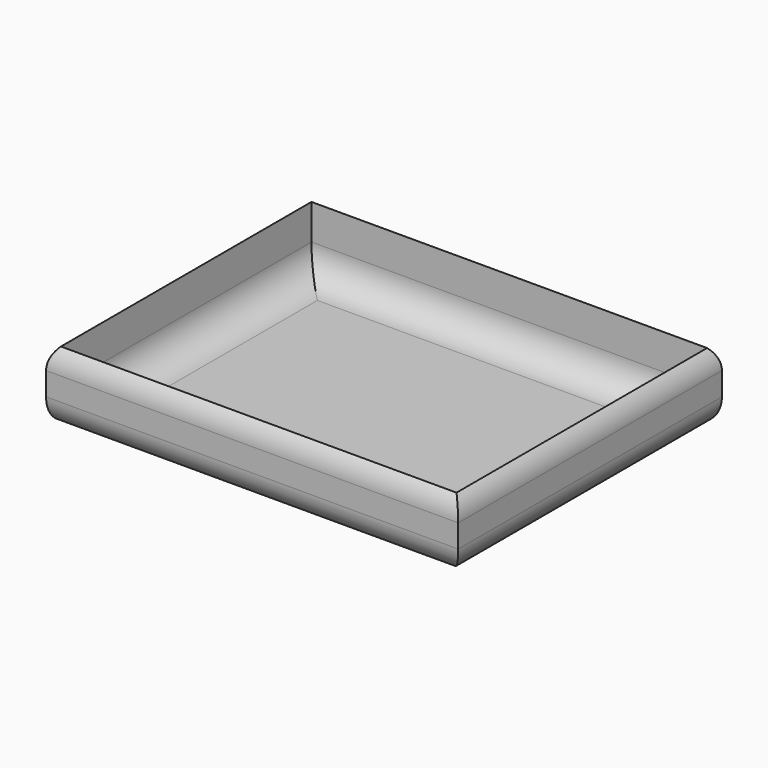
from build123d import *

# Parameters (mm, degrees)
F0_W        = 125
F0_H        = 100
F1_DEPTH    = 25
F2_T        = -2.5
F3_T1_DEPTH = 95
F3_T3_DEPTH = 120
F3_T5_DEPTH = 170
F3_T7_DEPTH = 145


# Not quite as in the source:
# - a fillet or chamfer that OpenCascade refuses, or shapes differently, is made with other operations: its cross-section is extruded or revolved along the edge and cut away or added


with BuildPart() as f1:
    # F0 (on Top) → F1 (new body)
    with BuildSketch(Plane.XY):
        with Locations((62.5, 50)):
            Rectangle(F0_W, F0_H)
    extrude(amount=F1_DEPTH)

    # F2
    f2_openings = [f1.faces().sort_by_distance(p)[0] for p in [
        (62.5, 50, 25),
    ]]
    offset(amount=F2_T, openings=f2_openings)

    # F3: fillet of radius 9 on 10 edges, made by hand

    # F3_s2 → F3_t1 (join)
    with BuildSketch(Plane.XZ.offset(-97.5)):
        with BuildLine():
            ThreePointArc((2.5, 11.5), (5.1360389693, 5.1360389693), (11.5, 2.5))
            Line((11.5, 2.5), (2.5, 2.5))
            Line((2.5, 2.5), (2.5, 11.5))
        make_face()
        with BuildLine():
            ThreePointArc((122.5, 11.5), (119.8639610307, 5.1360389693), (113.5, 2.5))
            Line((113.5, 2.5), (122.5, 2.5))
            Line((122.5, 2.5), (122.5, 11.5))
        make_face()
    extrude(amount=F3_T1_DEPTH)

    # F3_s4 → F3_t3 (join)
    with BuildSketch(Plane.YZ.offset(2.5)):
        with BuildLine():
            ThreePointArc((2.5, 11.5), (5.1360389693, 5.1360389693), (11.5, 2.5))
            Line((11.5, 2.5), (2.5, 2.5))
            Line((2.5, 2.5), (2.5, 11.5))
        make_face()
        with BuildLine():
            ThreePointArc((97.5, 11.5), (94.8639610307, 5.1360389693), (88.5, 2.5))
            Line((88.5, 2.5), (97.5, 2.5))
            Line((97.5, 2.5), (97.5, 11.5))
        make_face()
    extrude(amount=F3_T3_DEPTH)

    # F3_s6 → F3_t5 (cut)
    with BuildSketch(Plane.YZ.offset(-22.5)):
        with BuildLine():
            ThreePointArc((0, 16), (2.6360389693, 22.3639610307), (9, 25))
            Line((9, 25), (0, 25))
            Line((0, 25), (0, 16))
        make_face()
        with BuildLine():
            ThreePointArc((0, 9), (2.6360389693, 2.6360389693), (9, 0))
            Line((9, 0), (0, 0))
            Line((0, 0), (0, 9))
        make_face()
        with BuildLine():
            ThreePointArc((100, 16), (97.3639610307, 22.3639610307), (91, 25))
            Line((91, 25), (100, 25))
            Line((100, 25), (100, 16))
        make_face()
    extrude(amount=F3_T5_DEPTH, mode=Mode.SUBTRACT)

    # F3_s8 → F3_t7 (cut)
    with BuildSketch(Plane.XZ.offset(-122.5)):
        with BuildLine():
            ThreePointArc((116, 0), (122.3639610307, 2.6360389693), (125, 9))
            Line((125, 9), (125, 0))
            Line((125, 0), (116, 0))
        make_face()
        with BuildLine():
            ThreePointArc((116, 25), (122.3639610307, 22.3639610307), (125, 16))
            Line((125, 16), (125, 25))
            Line((125, 25), (116, 25))
        make_face()
        with BuildLine():
            ThreePointArc((0, 16), (2.6360389693, 22.3639610307), (9, 25))
            Line((9, 25), (0, 25))
            Line((0, 25), (0, 16))
        make_face()
    extrude(amount=F3_T7_DEPTH, mode=Mode.SUBTRACT)


solid = f1.part
